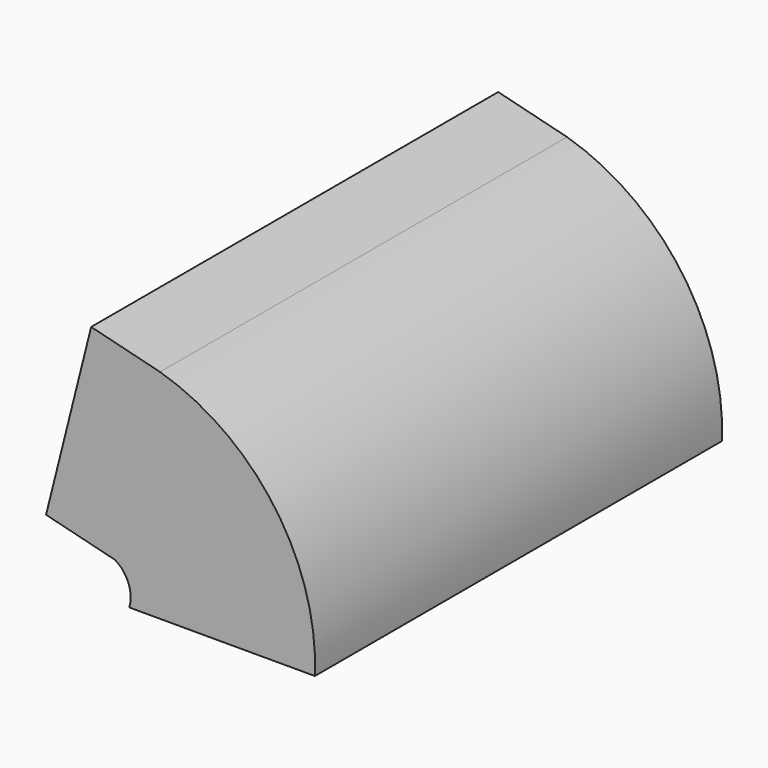
from build123d import *

# Parameters (mm, degrees)
F1_W     = 23.8884352148
F1_H     = 65.4788929969
F3_DEPTH = 9.144


with BuildPart() as f2:
    # F2: sweep along a path in F0
    with BuildLine(Plane.XZ) as f2_path:
        ThreePointArc((0, 0), (-5.1494897323, 17.4114904643), (-19.9215319008, 27.9691424221))
    # F1 (on Top) → F2 (sweep)
    with BuildSketch(Plane.XY):
        with Locations((-11.9442176074, 16.281622462)):
            Rectangle(F1_W, F1_H)
    sweep(path=f2_path.line)

    # F3 (add): a face of the model
    f3_faces = [f2.faces().sort_by_distance(p)[0] for p in [
        (-22.82294692, 16.281622462, 16.3826794096),
    ]]
    extrude(f3_faces, amount=F3_DEPTH)


solid = f2.part
